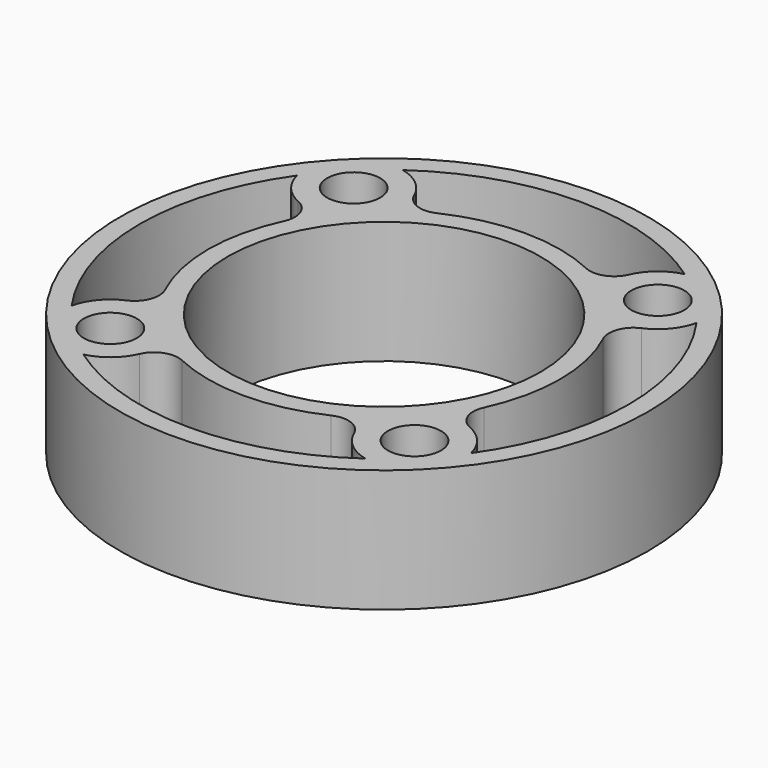
from build123d import *

# Parameters (mm, degrees)
F0_R            = 21.43125
F0_R_2          = 2.15265
F0_R_3          = 12.7
F1_DEPTH        = 9.9568
F3_DEPTH        = 9.9568
F3_COPIES_COUNT = 4
F4_R            = 1.984375


# Not quite as in the source:
# - a pattern or mirror of a feature is missing from the dataset's text; its kind, count and spacing are read off the source's solid


with BuildPart() as f1:
    # F0 (on Top) → F1 (new body)
    with BuildSketch(Plane.XY):
        Circle(F0_R)
        with Locations((-12.3478521665, -12.3478521665)):
            Circle(F0_R_2, mode=Mode.SUBTRACT)
        with Locations((12.3478521665, -12.3478521665)):
            Circle(F0_R_2, mode=Mode.SUBTRACT)
        with Locations((-12.3478521665, 12.3478521665)):
            Circle(F0_R_2, mode=Mode.SUBTRACT)
        Circle(F0_R_3, mode=Mode.SUBTRACT)
        with Locations((12.3478521665, 12.3478521665)):
            Circle(F0_R_2, mode=Mode.SUBTRACT)
    extrude(amount=F1_DEPTH)

    # F2 (on face) → F3 (cut, through all)
    with BuildSketch(Plane.XY.offset(9.9568)):
        with BuildLine():
            ThreePointArc((8.4692641257, 11.5067033254), (8.9929440308, 14.4681276118), (11.4430257563, 16.212081162))
            ThreePointArc((11.4430257563, 16.212081162), (0, 19.84375), (-11.4430257563, 16.212081162))
            ThreePointArc((-11.4430257563, 16.212081162), (-8.9929440308, 14.4681276118), (-8.4692641257, 11.5067033254))
            ThreePointArc((-8.4692641257, 11.5067033254), (0, 14.2875), (8.4692641257, 11.5067033254))
        make_face()
    f3 = extrude(amount=-F3_DEPTH, mode=Mode.SUBTRACT)

    # F3_copies: F3 ×4 about axis
    f3_copies_axis = Axis((0, 0, 0), (0, 0, 1))
    for i in range(1, F3_COPIES_COUNT):
        add(f3.rotate(f3_copies_axis, i * 360 / F3_COPIES_COUNT), mode=Mode.SUBTRACT)

    # F4
    f4_edges = [f1.edges().sort_by_distance(p)[0] for p in [
        (8.469264, 11.506703, 4.9784),
        (-8.469264, 11.506703, 4.9784),
        (8.469264, -11.506703, 4.9784),
        (-8.469264, -11.506703, 4.9784),
        (11.506703, 8.469264, 4.9784),
        (11.506703, -8.469264, 4.9784),
        (-11.506703, -8.469264, 4.9784),
        (-11.506703, 8.469264, 4.9784),
    ]]
    fillet(f4_edges, radius=F4_R)


solid = f1.part
